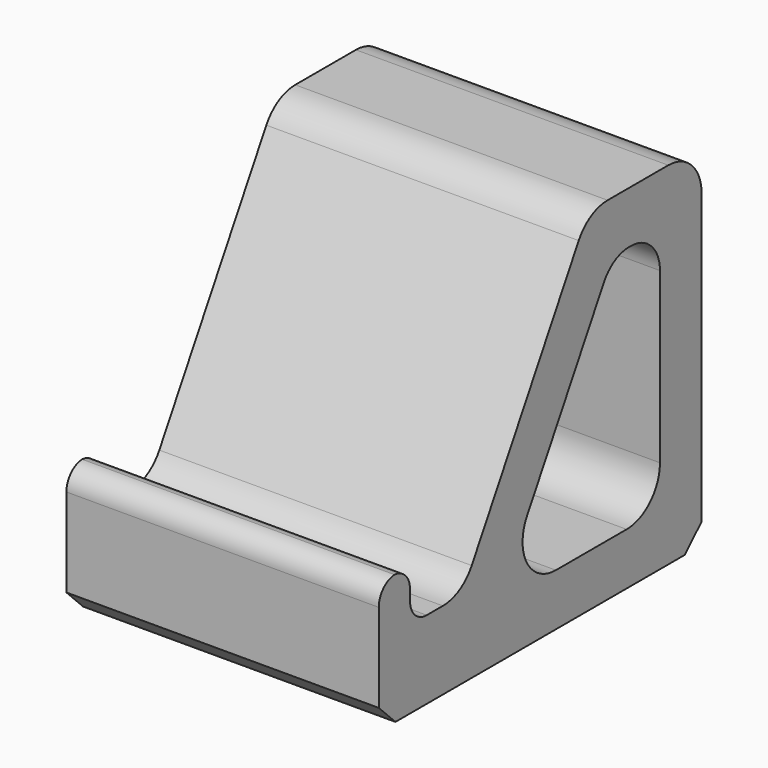
from build123d import *

# Parameters (mm, degrees)
F1_DEPTH    = 38.1
F3_DEPTH    = 76.2
F5_DEPTH    = 76.201
F6_T1_DEPTH = 76.2
F6_T3_DEPTH = 101.6
F7_R        = 10.16
F8_SIZE     = 5.08
F9_R        = 8.89


# Not quite as in the source:
# - a fillet or chamfer that OpenCascade refuses, or shapes differently, is made with other operations: its cross-section is extruded or revolved along the edge and cut away or added


with BuildPart() as f1:
    # F0 (on Right) → F1 (new body, symmetric)
    with BuildSketch(Plane.YZ):
        Polygon((-12.7, 31.75), (-12.7, 0), (12.7, 0), (56.6940905122, 76.2), (76.2, 76.2), (76.2, 0), (85.725, 0), (85.725, 85.725), (51.1948291982, 85.725), (12.7, 19.05), (7.200738686, 9.525), (-3.175, 9.525), (-3.175, 19.05), (-3.175, 31.75), align=None)
        Polygon((12.7, 19.05), (-3.175, 19.05), (-3.175, 9.525), (7.200738686, 9.525), align=None)
    extrude(amount=F1_DEPTH, both=True)

    # F2 (on face) → F3 (join, through all)
    with BuildSketch(Plane.YZ.offset(38.1)):
        Polygon((56.6940905122, 76.2), (12.7, 0), (76.2, 0), (76.2, 76.2), align=None)
    extrude(amount=-F3_DEPTH)

    # F4 (on face) → F5 (cut, through all)
    with BuildSketch(Plane.YZ.offset(38.1)):
        Polygon((58.5271776169, 73.025), (23.6985226281, 12.7), (73.025, 12.7), (73.025, 73.025), align=None)
    extrude(amount=-F5_DEPTH, mode=Mode.SUBTRACT)

    # F6: fillet of radius 5.08 on 3 edges, made by hand

    # F6_s2 → F6_t1 (join)
    with BuildSketch(Plane.YZ.offset(-38.1)):
        with BuildLine():
            ThreePointArc((-3.175, 24.13), (-1.6871024484, 20.5378975516), (1.905, 19.05))
            Line((1.905, 19.05), (-3.175, 19.05))
            Line((-3.175, 19.05), (-3.175, 24.13))
        make_face()
    extrude(amount=F6_T1_DEPTH)

    # F6_s4 → F6_t3 (cut)
    with BuildSketch(Plane.YZ.offset(-50.8)):
        with BuildLine():
            ThreePointArc((-3.175, 26.67), (-4.6628975516, 30.2621024484), (-8.255, 31.75))
            Line((-8.255, 31.75), (-3.175, 31.75))
            Line((-3.175, 31.75), (-3.175, 26.67))
        make_face()
        with BuildLine():
            ThreePointArc((-7.62, 31.75), (-11.2121024484, 30.2621024484), (-12.7, 26.67))
            Line((-12.7, 26.67), (-12.7, 31.75))
            Line((-12.7, 31.75), (-7.62, 31.75))
        make_face()
    extrude(amount=F6_T3_DEPTH, mode=Mode.SUBTRACT)

    # F7
    f7_edges = [f1.edges().sort_by_distance(p)[0] for p in [
        (0, 12.7, 19.05),
        (0, 51.194829, 85.725),
        (0, 85.725, 85.725),
        (0, 23.698523, 12.7),
        (0, 73.025, 12.7),
    ]]
    fillet(f7_edges, radius=F7_R)

    # F8
    f8_edges = [f1.edges().sort_by_distance(p)[0] for p in [
        (0, 85.725, 0),
        (0, -12.7, 0),
    ]]
    chamfer(f8_edges, length=F8_SIZE)

    # F9
    f9_edges = [f1.edges().sort_by_distance(p)[0] for p in [
        (0, 73.025, 73.025),
        (0, 58.527178, 73.025),
    ]]
    fillet(f9_edges, radius=F9_R)


solid = f1.part
